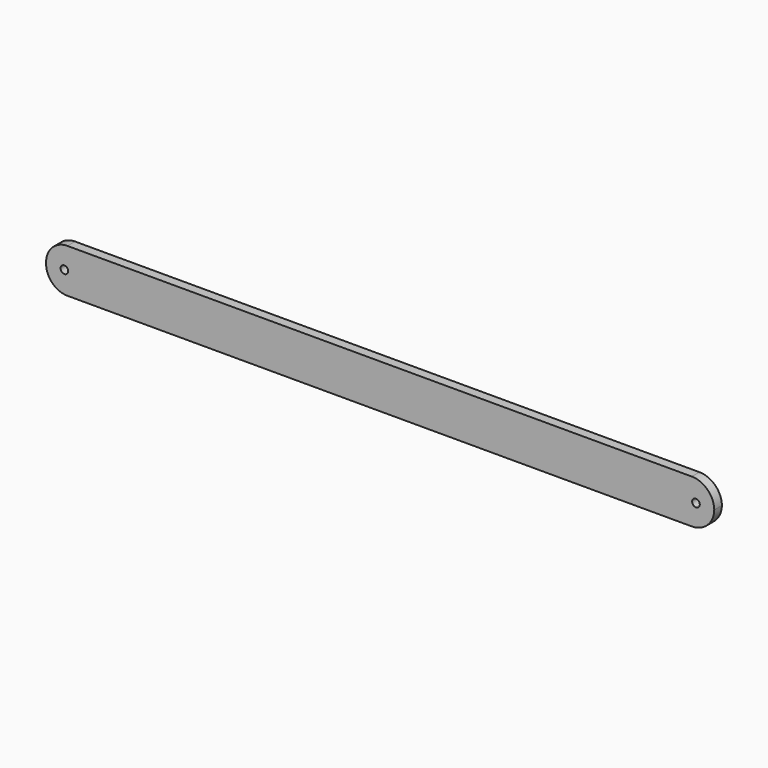
from build123d import *

# Parameters (mm, degrees)
F0_W        = 111.125
F0_H        = 7.3025
F0_R        = 0.635
F1_DEPTH    = 1.5875
F2_R        = 3.5566194201
F3_T1_DEPTH = 20.2904124677


# Not quite as in the source:
# - a fillet or chamfer that OpenCascade refuses, or shapes differently, is made with other operations: its cross-section is extruded or revolved along the edge and cut away or added


with BuildPart() as f1:
    # F0 (on Front) → F1 (new body)
    with BuildSketch(Plane.XZ):
        with Locations((8.7715025485, 10.1259618964)):
            Rectangle(F0_W, F0_H)
        with Locations((-43.7429974515, 10.1259618964)):
            Circle(F0_R, mode=Mode.SUBTRACT)
        with Locations((61.2860025485, 10.1196118964)):
            Circle(F0_R, mode=Mode.SUBTRACT)
    extrude(amount=F1_DEPTH)

    # F2
    f2_edges = [f1.edges().sort_by_distance(p)[0] for p in [
        (-46.790997, -0.79375, 13.777212),
        (-46.790997, -0.79375, 6.474712),
    ]]
    fillet(f2_edges, radius=F2_R)

    # F3: fillet of radius 3.7405824935 on 2 edges, made by hand

    # F3_s2 → F3_t1 (cut)
    with BuildSketch(Plane.XZ.offset(-9.3514562339)):
        with BuildLine():
            ThreePointArc((60.5934200549, 13.7772118964), (63.2384113017, 12.6816206496), (64.3340025485, 10.0366294028))
            Line((64.3340025485, 10.0366294028), (64.3340025485, 13.7772118964))
            Line((64.3340025485, 13.7772118964), (60.5934200549, 13.7772118964))
        make_face()
        with BuildLine():
            ThreePointArc((64.3340025485, 10.2152943899), (63.2384113017, 7.5703031432), (60.5934200549, 6.4747118964))
            Line((60.5934200549, 6.4747118964), (64.3340025485, 6.4747118964))
            Line((64.3340025485, 6.4747118964), (64.3340025485, 10.2152943899))
        make_face()
    extrude(amount=F3_T1_DEPTH, mode=Mode.SUBTRACT)


solid = f1.part
